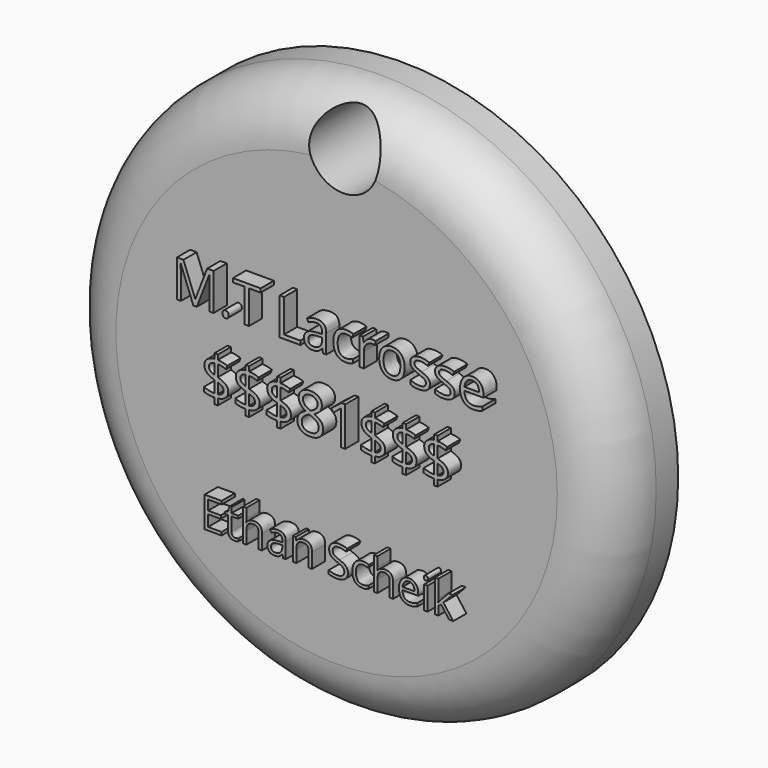
from build123d import *

# Parameters (mm, degrees)
F0_R           = 25.4844088121
F1_DEPTH       = 7.62
F2_R           = 3.2108352297
F3_DEPTH       = 22.606
F4_TEXT_SIZE   = 4.7947331849
F4_TEXT_SIZE_2 = 3.9486059298
F5_DEPTH       = 1.524
F7_TEXT_SIZE   = 5.0767790526
F8_DEPTH       = 1.524


# Not quite as in the source:
# - a fillet or chamfer that OpenCascade refuses, or shapes differently, is made with other operations: its cross-section is extruded or revolved along the edge and cut away or added
# - Text() gives the source's letters only with a copy of the font that has no kerning and outlines rounded to 1/6400 em; it was checked with that copy


with BuildPart() as f1:
    # F0 (on Front) → F1 (new body)
    with BuildSketch(Plane.XZ):
        with Locations((20.6117127091, 43.558742851)):
            Circle(F0_R)
    extrude(amount=F1_DEPTH)

    # F2 (on face) → F3 (cut)
    with BuildSketch(Plane.XZ.offset(7.62)):
        with Locations((21.220928058, 64.8812055588)):
            Circle(F2_R)
    extrude(amount=-F3_DEPTH, mode=Mode.SUBTRACT)

    # F4 (on face) → F5 (join)
    with BuildSketch(Plane.XZ.offset(7.62)):
        with Locations((6.5998081118, 49.0416660905)):
            Text('M.T Lacrosse', F4_TEXT_SIZE, font='Open Sans', text_align=(TextAlign.LEFT, TextAlign.BOTTOM))
        with Locations((9.2397304252, 31.1714075506)):
            Text('Ethan Scheik', F4_TEXT_SIZE_2, font='Open Sans', text_align=(TextAlign.LEFT, TextAlign.BOTTOM))
    extrude(amount=F5_DEPTH)

    # F6: fillet of radius 5.08 on 1 edges, made by hand

    # F6_s1 → F6_t2 (revolve, cut)
    with BuildSketch(Plane.XY.offset(43.558742851)):
        with BuildLine():
            ThreePointArc((46.0961215212, -2.54), (44.6082239696, -6.1321024484), (41.0161215212, -7.62))
            Line((41.0161215212, -7.62), (46.0961215212, -7.62))
            Line((46.0961215212, -7.62), (46.0961215212, -2.54))
        make_face()
    revolve(axis=Axis((20.6117127091, -7.62, 43.558742851), (0, -1, 0)), mode=Mode.SUBTRACT)

    # F7 (on face) → F8 (join)
    with BuildSketch(Plane.XZ.offset(7.62)):
        with Locations((9.2397341505, 41.9341772795)):
            Text('$$$81$$$', F7_TEXT_SIZE, font='Open Sans', text_align=(TextAlign.LEFT, TextAlign.BOTTOM))
    extrude(amount=F8_DEPTH)


solid = f1.part
